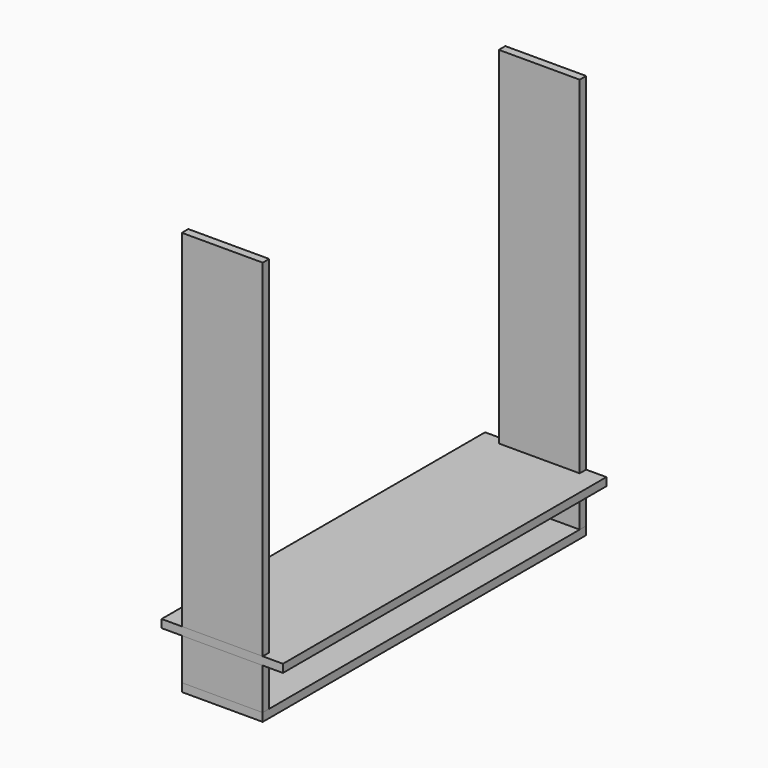
from build123d import *

# Parameters (mm, degrees)
F0_W     = 200
F0_H     = 20
F1_DEPTH = 1000
F2_W     = 200
F2_H     = 20.362149924
F3_DEPTH = 1000
F4_DEPTH = 1000


with BuildPart() as f1:
    # F0 (on Top) → F1 (new body)
    with BuildSketch(Plane.XY):
        with Locations((100, 10)):
            Rectangle(F0_W, F0_H)
    extrude(amount=F1_DEPTH)

    # F2 (on face) → F3 (join)
    with BuildSketch(Plane.XZ):
        with Locations((100, 10.181074962)):
            Rectangle(F2_W, F2_H)
    extrude(amount=-F3_DEPTH)


with BuildPart() as f1b:
    # F0 (on Top) → F1, piece 2 (new body)
    with BuildSketch(Plane.XY):
        with Locations((100, 990)):
            Rectangle(F0_W, F0_H)
    extrude(amount=F1_DEPTH)


with BuildPart() as f4:
    # F2 (on face) → F4 (new body)
    with BuildSketch(Plane.XZ):
        with Locations((100, 10.181074962)):
            Rectangle(F2_W, F2_H)
    extrude(amount=-F4_DEPTH)


with BuildPart() as f4b:
    # F2 (on face) → F4, piece 2 (new body)
    with BuildSketch(Plane.XZ):
        Polygon((-50, 122.862149924), (0, 122.862149924), (250, 122.862149924), (250, 142.862149924), (-50, 142.862149924), align=None)
    extrude(amount=-F4_DEPTH)


solid = Compound([f1.part, f1b.part, f4.part, f4b.part])
